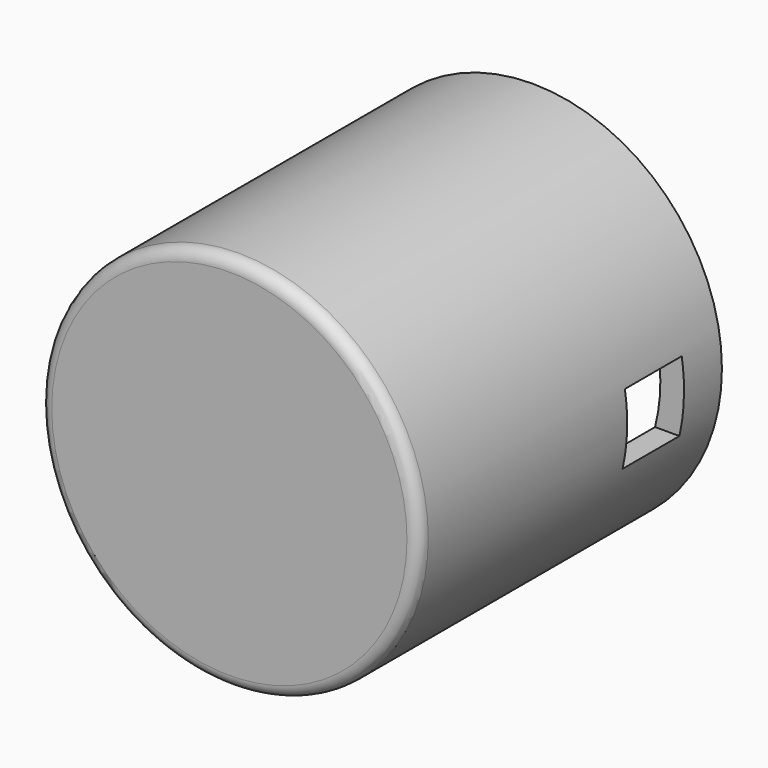
from build123d import *

# Parameters (mm, degrees)
F0_R          = 16
F0_R_2        = 14
F1_DEPTH      = 32
F2_R          = 14
F3_DEPTH      = 30
F4_R          = 1
F5_W          = 6
F5_H          = 6
F6_DEPTH      = 35.5
F6_DEPTH_BACK = 16.5


# Not quite as in the source:
# - a feature names something its author has since deleted; it is built from what else it names


with BuildPart() as f1:
    # F0 (on Front) → F1 (new body)
    with BuildSketch(Plane.XZ):
        with Locations((-13.5661968961, 9.2302449048)):
            Circle(F0_R)
        with Locations((-13.5661968961, 9.2302449048)):
            Circle(F0_R_2, mode=Mode.SUBTRACT)
        with Locations((-13.5661968961, 9.2302449048)):
            Circle(F0_R_2)
    extrude(amount=F1_DEPTH)

    # F2 (on face) → F3 (cut)
    with BuildSketch(Plane(origin=(0, 0, 0), x_dir=(-1, 0, 0), z_dir=(0, 1, 0))):
        with Locations((13.5661968961, 9.2302449048)):
            Circle(F2_R)
    extrude(amount=-F3_DEPTH, mode=Mode.SUBTRACT)

    # F4
    f4_edges = [f1.edges().sort_by_distance(p)[0] for p in [
        (-29.566197, -32, 9.230245),
    ]]
    fillet(f4_edges, radius=F4_R)

    # F5 (on Right) → F6 (cut, two sides)
    with BuildSketch(Plane.YZ) as f6_sk:
        with Locations((-7, 8.7253677193)):
            Rectangle(F5_W, F5_H)
    extrude(amount=-F6_DEPTH, mode=Mode.SUBTRACT)
    extrude(f6_sk.sketch, amount=F6_DEPTH_BACK, mode=Mode.SUBTRACT)


solid = f1.part
